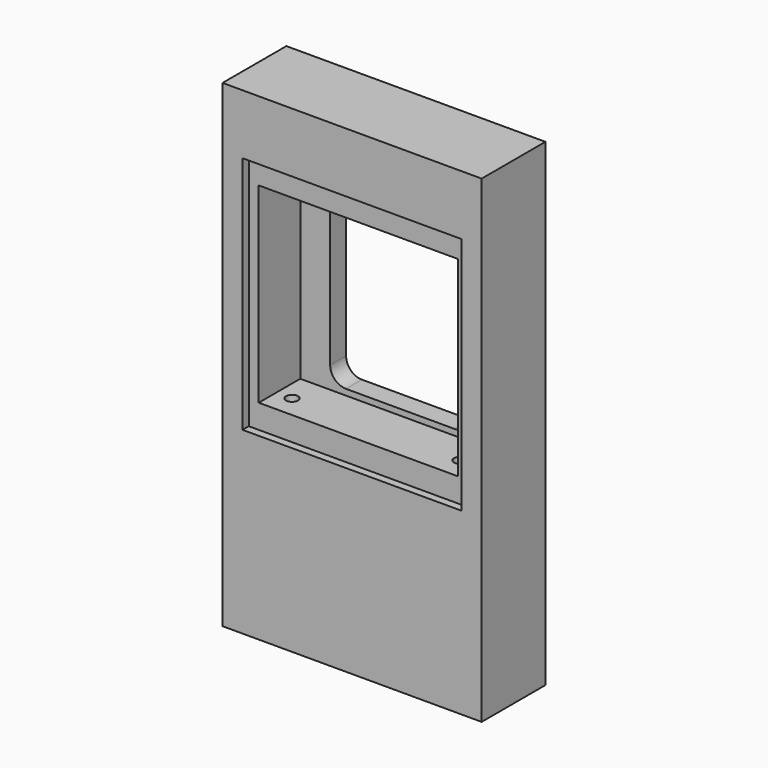
from build123d import *

# Parameters (mm, degrees)
F0_W     = 165.1
F0_H     = 304.8
F0_W_2   = 139.7
F0_H_2   = 152.4
F0_W_3   = 127
F0_H_3   = 121.92
F0_W_4   = 88.9
F0_H_4   = 114.3
F1_DEPTH = 50.8
F2_DEPTH = 5
F3_DEPTH = 38.1
F4_R     = 10
F5_R     = 3.81
F6_DEPTH = 129.54


# Not quite as in the source:
# - a feature names something its author has since deleted; it is built from what else it names


with BuildPart() as f1:
    # F0 (on Front) → F1 (new body)
    with BuildSketch(Plane.XZ):
        with Locations((0, -38.1)):
            Rectangle(F0_W, F0_H)
        Rectangle(F0_W_2, F0_H_2, mode=Mode.SUBTRACT)
        Rectangle(F0_W_2, F0_H_2)
        Rectangle(F0_W_3, F0_H_3, mode=Mode.SUBTRACT)
        Rectangle(F0_W_3, F0_H_3)
        Rectangle(F0_W_4, F0_H_4, mode=Mode.SUBTRACT)
    extrude(amount=-F1_DEPTH)

    # F0 (on Front) → F2 (cut)
    with BuildSketch(Plane.XZ):
        Rectangle(F0_W_2, F0_H_2)
        Rectangle(F0_W_3, F0_H_3, mode=Mode.SUBTRACT)
    extrude(amount=-F2_DEPTH, mode=Mode.SUBTRACT)

    # F0 (on Front) → F3 (cut)
    with BuildSketch(Plane.XZ):
        Rectangle(F0_W_3, F0_H_3)
        Rectangle(F0_W_4, F0_H_4, mode=Mode.SUBTRACT)
    extrude(amount=-F3_DEPTH, mode=Mode.SUBTRACT)

    # F4
    f4_edges = [f1.edges().sort_by_distance(p)[0] for p in [
        (-44.45, 44.45, 57.15),
        (44.45, 44.45, 57.15),
        (-44.45, 44.45, -57.15),
        (44.45, 44.45, -57.15),
    ]]
    fillet(f4_edges, radius=F4_R)

    # F5 (on face) → F6 (cut, through all)
    with BuildSketch(Plane.XY.offset(-60.96)):
        with Locations((-53.5, 19.05)):
            Circle(F5_R)
        with Locations((53.4924, 19.05)):
            Circle(F5_R)
    extrude(amount=-F6_DEPTH, mode=Mode.SUBTRACT)


solid = f1.part
